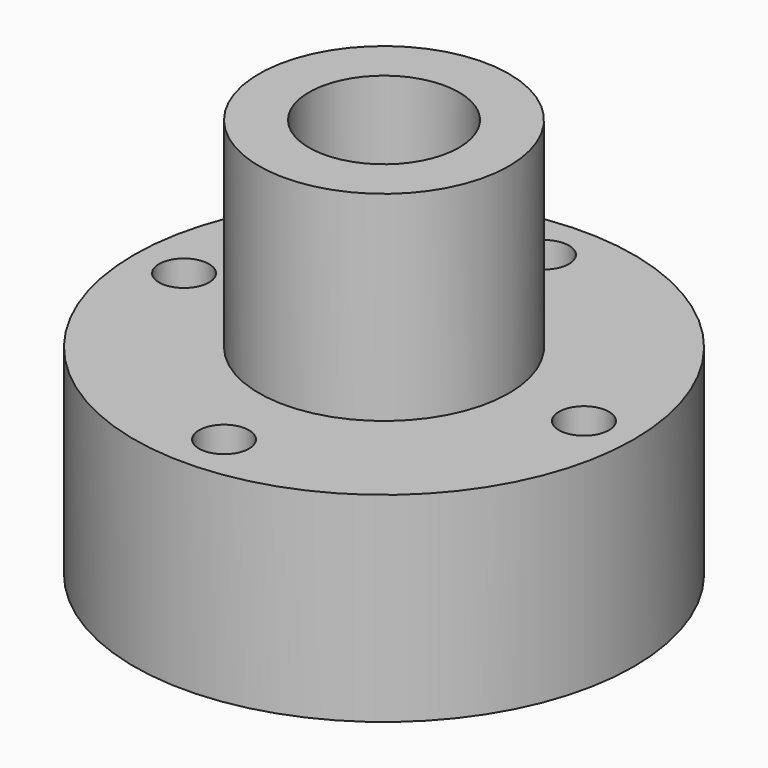
from build123d import *

# Parameters (mm, degrees)
F0_R            = 15.875
F0_R_2          = 7.9375
F0_R_3          = 4.7625
F1_DEPTH        = 12.7
F2_DEPTH        = 25.4
F3_R            = 1.5875
F4_DEPTH        = 12.7
F4_COPIES_COUNT = 4


# Not quite as in the source:
# - a pattern or mirror of a feature is missing from the dataset's text; its kind, count and spacing are read off the source's solid


with BuildPart() as f1:
    # F0 (on Top) → F1 (new body)
    with BuildSketch(Plane.XY):
        Circle(F0_R)
        Circle(F0_R_2, mode=Mode.SUBTRACT)
        Circle(F0_R_2)
        Circle(F0_R_3, mode=Mode.SUBTRACT)
    extrude(amount=F1_DEPTH)

    # F0 (on Top) → F2 (join)
    with BuildSketch(Plane.XY):
        Circle(F0_R_2)
        Circle(F0_R_3, mode=Mode.SUBTRACT)
    extrude(amount=F2_DEPTH)

    # F3 (on face) → F4 (cut)
    with BuildSketch(Plane.XY.offset(12.7)):
        with Locations((0, 12.7)):
            Circle(F3_R)
    f4 = extrude(amount=-F4_DEPTH, mode=Mode.SUBTRACT)

    # F4_copies: F4 ×4 about axis
    f4_copies_axis = Axis((0, 0, 0), (0, 0, 1))
    for i in range(1, F4_COPIES_COUNT):
        add(f4.rotate(f4_copies_axis, i * 360 / F4_COPIES_COUNT), mode=Mode.SUBTRACT)


solid = f1.part
